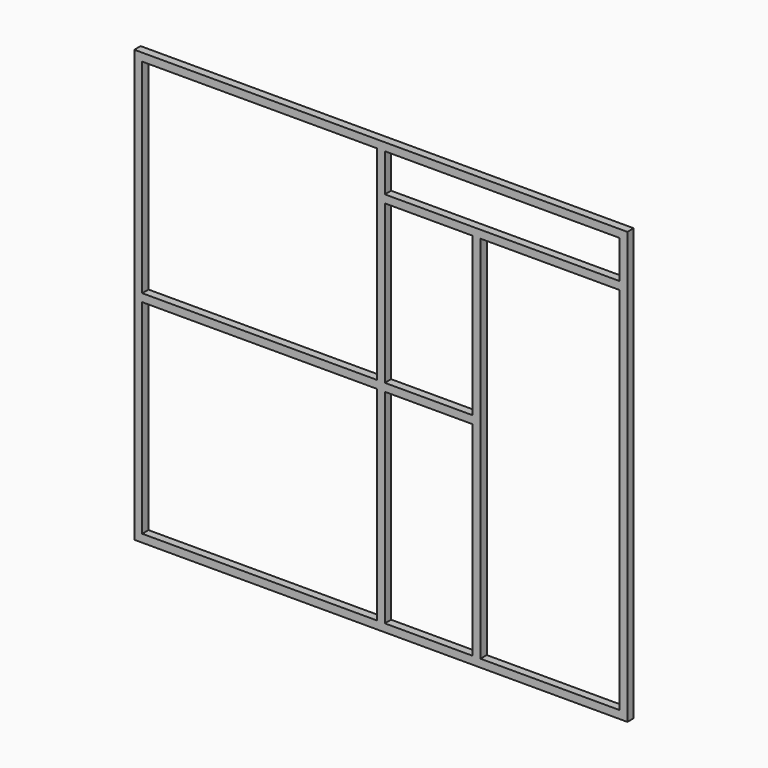
from build123d import *

# Parameters (mm, degrees)
F0_W     = 2000
F0_H     = 1750
F0_W_2   = 952
F0_H_2   = 32
F0_W_3   = 32
F0_H_3   = 827
F0_W_4   = 356
F1_DEPTH = 32


# Not quite as in the source:
# - a feature names something its author has since deleted; it is built from what else it names


with BuildPart() as f1:
    # F0 (on Front) → F1 (new body)
    with BuildSketch(Plane.XZ):
        with Locations((1000, 875)):
            Rectangle(F0_W, F0_H)
        Polygon((984, 32), (32, 32), (32, 859), (32, 891), (32, 1718), (984, 1718), (1016, 1718), (1968, 1718), (1968, 1564), (1968, 1532), (1968, 891), (1968, 859), (1968, 32), (1404, 32), (1372, 32), (1016, 32), align=None, mode=Mode.SUBTRACT)
        with Locations((508, 875)):
            Rectangle(F0_W_2, F0_H_2)
        with Locations((1000, 445.5)):
            Rectangle(F0_W_3, F0_H_3)
        with Locations((1000, 875)):
            Rectangle(F0_W_3, F0_H_2)
        Polygon((984, 1718), (984, 891), (1016, 891), (1016, 1532), (1016, 1564), (1016, 1718), align=None)
        with Locations((1194, 875)):
            Rectangle(F0_W_4, F0_H_2)
        Polygon((1372, 859), (1372, 32), (1404, 32), (1404, 1532), (1372, 1532), (1372, 891), align=None)
        Polygon((1016, 1564), (1016, 1532), (1372, 1532), (1404, 1532), (1968, 1532), (1968, 1564), align=None)
    extrude(amount=F1_DEPTH)


solid = f1.part
